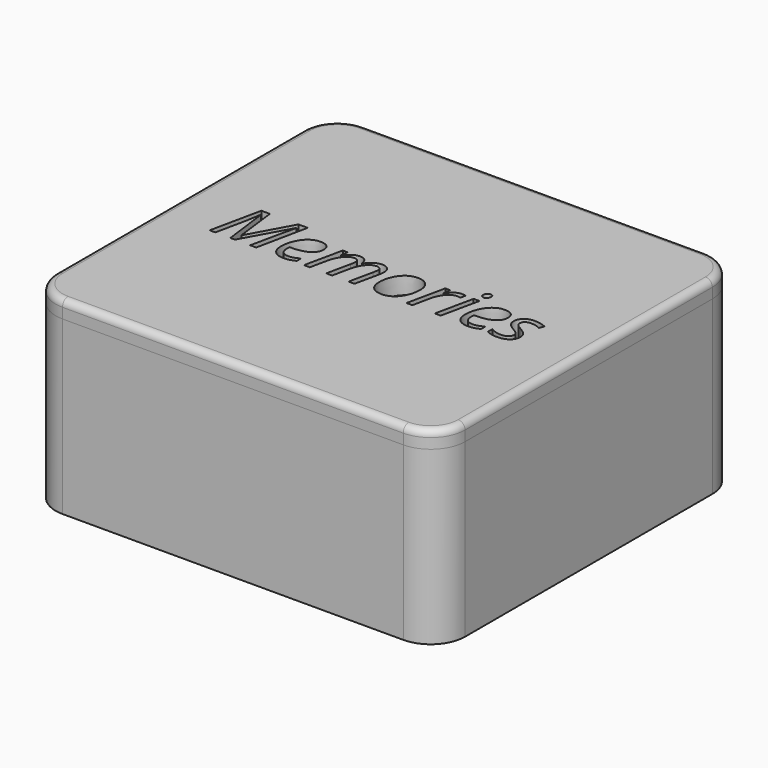
from build123d import *

# Parameters (mm, degrees)
F0_W         = 119.22
F0_H         = 110
F0_W_2       = 109.22
F0_H_2       = 100
F1_DEPTH     = 5
F2_DEPTH     = 45
F3_R         = 5
F4_R         = 10
F6_DEPTH     = 5
F7_DEPTH     = 10
F8_R         = 2
F8_2_R       = 2
F9_TEXT_SIZE = 20.8333333333
F10_DEPTH    = 25
F11_R        = 2


# Not quite as in the source:
# - Text() gives the source's letters only with a copy of the font that has no kerning and outlines rounded to 1/6400 em; it was checked with that copy


with BuildPart() as f1:
    # F0 (on Top) → F1 (new body)
    with BuildSketch(Plane.XY):
        Rectangle(F0_W, F0_H)
        Rectangle(F0_W_2, F0_H_2, mode=Mode.SUBTRACT)
        Rectangle(F0_W_2, F0_H_2)
    extrude(amount=-F1_DEPTH)

    # F0 (on Top) → F2 (join)
    with BuildSketch(Plane.XY):
        Rectangle(F0_W, F0_H)
        Rectangle(F0_W_2, F0_H_2, mode=Mode.SUBTRACT)
    extrude(amount=F2_DEPTH)

    # F3
    f3_edges = [f1.edges().sort_by_distance(p)[0] for p in [
        (-54.61, 50, 22.5),
        (54.61, 50, 22.5),
        (54.61, -50, 22.5),
        (-54.61, -50, 22.5),
    ]]
    fillet(f3_edges, radius=F3_R)

    # F4
    f4_edges = [f1.edges().sort_by_distance(p)[0] for p in [
        (-59.61, -55, 20),
        (59.61, -55, 20),
        (59.61, 55, 20),
        (-59.61, 55, 20),
    ]]
    fillet(f4_edges, radius=F4_R)

    # F8
    f8_edges = [f1.edges().sort_by_distance(p)[0] for p in [
        (-54.61, 0, 45),
    ]]
    fillet(f8_edges, radius=F8_R)


with BuildPart() as f6:
    # F5 (on face) → F6 (new body)
    with BuildSketch(Plane.XY.offset(45)):
        with BuildLine():
            Line((-59.61, 45), (-59.61, -45))
            ThreePointArc((-59.61, -45), (-56.6810678119, -52.0710678119), (-49.61, -55))
            Line((-49.61, -55), (49.61, -55))
            ThreePointArc((49.61, -55), (56.6810678119, -52.0710678119), (59.61, -45))
            Line((59.61, -45), (59.61, 45))
            ThreePointArc((59.61, 45), (56.6810678119, 52.0710678119), (49.61, 55))
            Line((49.61, 55), (-49.61, 55))
            ThreePointArc((-49.61, 55), (-56.6810678119, 52.0710678119), (-59.61, 45))
        make_face()
        with BuildLine():
            ThreePointArc((54.61, -45), (53.1455339059, -48.5355339059), (49.61, -50))
            Line((49.61, -50), (-49.61, -50))
            ThreePointArc((-49.61, -50), (-53.1455339059, -48.5355339059), (-54.61, -45))
            Line((-54.61, -45), (-54.61, 45))
            ThreePointArc((-54.61, 45), (-53.1455339059, 48.5355339059), (-49.61, 50))
            Line((-49.61, 50), (49.61, 50))
            ThreePointArc((49.61, 50), (53.1455339059, 48.5355339059), (54.61, 45))
            Line((54.61, 45), (54.61, -45))
        make_face(mode=Mode.SUBTRACT)
        with BuildLine():
            Line((-49.61, -50), (49.61, -50))
            ThreePointArc((49.61, -50), (53.1455339059, -48.5355339059), (54.61, -45))
            Line((54.61, -45), (54.61, 45))
            ThreePointArc((54.61, 45), (53.1455339059, 48.5355339059), (49.61, 50))
            Line((49.61, 50), (-49.61, 50))
            ThreePointArc((-49.61, 50), (-53.1455339059, 48.5355339059), (-54.61, 45))
            Line((-54.61, 45), (-54.61, -45))
            ThreePointArc((-54.61, -45), (-53.1455339059, -48.5355339059), (-49.61, -50))
        make_face()
        with BuildLine():
            ThreePointArc((-49.61, -49.5), (-52.7919805153, -48.1819805153), (-54.11, -45))
            Line((-54.11, -45), (-54.11, 45))
            ThreePointArc((-54.11, 45), (-52.7919805153, 48.1819805153), (-49.61, 49.5))
            Line((-49.61, 49.5), (49.61, 49.5))
            ThreePointArc((49.61, 49.5), (52.7919805153, 48.1819805153), (54.11, 45))
            Line((54.11, 45), (54.11, -45))
            ThreePointArc((54.11, -45), (52.7919805153, -48.1819805153), (49.61, -49.5))
            Line((49.61, -49.5), (-49.61, -49.5))
        make_face(mode=Mode.SUBTRACT)
        with BuildLine():
            Line((-54.11, 45), (-54.11, -45))
            ThreePointArc((-54.11, -45), (-52.7919805153, -48.1819805153), (-49.61, -49.5))
            Line((-49.61, -49.5), (49.61, -49.5))
            ThreePointArc((49.61, -49.5), (52.7919805153, -48.1819805153), (54.11, -45))
            Line((54.11, -45), (54.11, 45))
            ThreePointArc((54.11, 45), (52.7919805153, 48.1819805153), (49.61, 49.5))
            Line((49.61, 49.5), (-49.61, 49.5))
            ThreePointArc((-49.61, 49.5), (-52.7919805153, 48.1819805153), (-54.11, 45))
        make_face()
        with BuildLine():
            ThreePointArc((-49.61, -47), (-51.0242135624, -46.4142135624), (-51.61, -45))
            Line((-51.61, -45), (-51.61, 45))
            ThreePointArc((-51.61, 45), (-51.0242135624, 46.4142135624), (-49.61, 47))
            Line((-49.61, 47), (49.61, 47))
            ThreePointArc((49.61, 47), (51.0242135624, 46.4142135624), (51.61, 45))
            Line((51.61, 45), (51.61, -45))
            ThreePointArc((51.61, -45), (51.0242135624, -46.4142135624), (49.61, -47))
            Line((49.61, -47), (-49.61, -47))
        make_face(mode=Mode.SUBTRACT)
        with BuildLine():
            Line((-51.61, 45), (-51.61, -45))
            ThreePointArc((-51.61, -45), (-51.0242135624, -46.4142135624), (-49.61, -47))
            Line((-49.61, -47), (49.61, -47))
            ThreePointArc((49.61, -47), (51.0242135624, -46.4142135624), (51.61, -45))
            Line((51.61, -45), (51.61, 45))
            ThreePointArc((51.61, 45), (51.0242135624, 46.4142135624), (49.61, 47))
            Line((49.61, 47), (-49.61, 47))
            ThreePointArc((-49.61, 47), (-51.0242135624, 46.4142135624), (-51.61, 45))
        make_face()
    extrude(amount=F6_DEPTH)

    # F5 (on face) → F7 (join)
    with BuildSketch(Plane.XY.offset(45)):
        with BuildLine():
            Line((-54.11, 45), (-54.11, -45))
            ThreePointArc((-54.11, -45), (-52.7919805153, -48.1819805153), (-49.61, -49.5))
            Line((-49.61, -49.5), (49.61, -49.5))
            ThreePointArc((49.61, -49.5), (52.7919805153, -48.1819805153), (54.11, -45))
            Line((54.11, -45), (54.11, 45))
            ThreePointArc((54.11, 45), (52.7919805153, 48.1819805153), (49.61, 49.5))
            Line((49.61, 49.5), (-49.61, 49.5))
            ThreePointArc((-49.61, 49.5), (-52.7919805153, 48.1819805153), (-54.11, 45))
        make_face()
        with BuildLine():
            ThreePointArc((-49.61, -47), (-51.0242135624, -46.4142135624), (-51.61, -45))
            Line((-51.61, -45), (-51.61, 45))
            ThreePointArc((-51.61, 45), (-51.0242135624, 46.4142135624), (-49.61, 47))
            Line((-49.61, 47), (49.61, 47))
            ThreePointArc((49.61, 47), (51.0242135624, 46.4142135624), (51.61, 45))
            Line((51.61, 45), (51.61, -45))
            ThreePointArc((51.61, -45), (51.0242135624, -46.4142135624), (49.61, -47))
            Line((49.61, -47), (-49.61, -47))
        make_face(mode=Mode.SUBTRACT)
    extrude(amount=-F7_DEPTH)

    # F8#2
    f8_2_edges = [f6.edges().sort_by_distance(p)[0] for p in [
        (-54.11, 0, 45),
        (-51.61, 0, 45),
    ]]
    fillet(f8_2_edges, radius=F8_2_R)

    # F9 (on face) → F10 (cut)
    with BuildSketch(Plane.XY.offset(50)):
        with Locations((-45.6168619792, -7.5)):
            Text('Memories', F9_TEXT_SIZE, font='Open Sans', font_style=FontStyle.ITALIC, text_align=(TextAlign.LEFT, TextAlign.BOTTOM))
        with BuildLine():
            add(Edge.make_bspline(
                [(-20.5973307292, 2.0426432292), (-20.9684244792, 2.3990885417), (-21.7626953125, 2.3990885417)],
                knots=[0, 0, 0, 1, 1, 1], degree=2))
            add(Edge.make_bspline(
                [(-21.7626953125, 2.3990885417), (-22.8108723958, 2.3990885417), (-23.7320963542, 1.4420572917)],
                knots=[0, 0, 0, 1, 1, 1], degree=2))
            add(Edge.make_bspline(
                [(-23.7320963542, 1.4420572917), (-24.6533203125, 0.4850260417), (-25.1416015625, -1.2141927083)],
                knots=[0, 0, 0, 1, 1, 1], degree=2))
            Line((-25.1416015625, -1.2141927083), (-25.0179036458, -1.2141927083))
            add(Edge.make_bspline(
                [(-25.0179036458, -1.2141927083), (-22.7001953125, -1.2141927083), (-21.4632161458, -0.6087239583)],
                knots=[0, 0, 0, 1, 1, 1], degree=2))
            add(Edge.make_bspline(
                [(-21.4632161458, -0.6087239583), (-20.2262369792, -0.0032552083), (-20.2262369792, 1.1458333333)],
                knots=[0, 0, 0, 1, 1, 1], degree=2))
            add(Edge.make_bspline(
                [(-20.2262369792, 1.1458333333), (-20.2262369792, 1.6861979167), (-20.5973307292, 2.0426432292)],
                knots=[0, 0, 0, 1, 1, 1], degree=2))
        make_face()
        with BuildLine():
            add(Edge.make_bspline(
                [(8.7272135417, -3.3951822917), (9.2008463542, -2.0279947917), (9.2008463542, -0.2669270833)],
                knots=[0, 0, 0, 1, 1, 1], degree=2))
            add(Edge.make_bspline(
                [(9.2008463542, -0.2669270833), (9.2008463542, 0.9016927083), (8.564453125, 1.6292317708)],
                knots=[0, 0, 0, 1, 1, 1], degree=2))
            add(Edge.make_bspline(
                [(8.564453125, 1.6292317708), (7.9280598958, 2.3567708333), (6.8408203125, 2.3567708333)],
                knots=[0, 0, 0, 1, 1, 1], degree=2))
            add(Edge.make_bspline(
                [(6.8408203125, 2.3567708333), (5.7307942708, 2.3567708333), (4.8518880208, 1.6048177083)],
                knots=[0, 0, 0, 1, 1, 1], degree=2))
            add(Edge.make_bspline(
                [(4.8518880208, 1.6048177083), (3.9729817708, 0.8528645833), (3.4895833333, -0.4850260417)],
                knots=[0, 0, 0, 1, 1, 1], degree=2))
            add(Edge.make_bspline(
                [(3.4895833333, -0.4850260417), (3.0061848958, -1.8229166667), (3.0061848958, -3.4602864583)],
                knots=[0, 0, 0, 1, 1, 1], degree=2))
            add(Edge.make_bspline(
                [(3.0061848958, -3.4602864583), (3.0061848958, -4.794921875), (3.65234375, -5.5224609375)],
                knots=[0, 0, 0, 1, 1, 1], degree=2))
            add(Edge.make_bspline(
                [(3.65234375, -5.5224609375), (4.2985026042, -6.25), (5.5094401042, -6.25)],
                knots=[0, 0, 0, 1, 1, 1], degree=2))
            add(Edge.make_bspline(
                [(5.5094401042, -6.25), (6.5673828125, -6.25), (7.4104817708, -5.5061848958)],
                knots=[0, 0, 0, 1, 1, 1], degree=2))
            add(Edge.make_bspline(
                [(7.4104817708, -5.5061848958), (8.2535807292, -4.7623697917), (8.7272135417, -3.3951822917)],
                knots=[0, 0, 0, 1, 1, 1], degree=2))
        make_face()
        with BuildLine():
            add(Edge.make_bspline(
                [(33.0712890625, 2.0426432292), (32.7001953125, 2.3990885417), (31.9059244792, 2.3990885417)],
                knots=[0, 0, 0, 1, 1, 1], degree=2))
            add(Edge.make_bspline(
                [(31.9059244792, 2.3990885417), (30.8577473958, 2.3990885417), (29.9365234375, 1.4420572917)],
                knots=[0, 0, 0, 1, 1, 1], degree=2))
            add(Edge.make_bspline(
                [(29.9365234375, 1.4420572917), (29.0152994792, 0.4850260417), (28.5270182292, -1.2141927083)],
                knots=[0, 0, 0, 1, 1, 1], degree=2))
            Line((28.5270182292, -1.2141927083), (28.6507161458, -1.2141927083))
            add(Edge.make_bspline(
                [(28.6507161458, -1.2141927083), (30.9684244792, -1.2141927083), (32.2054036458, -0.6087239583)],
                knots=[0, 0, 0, 1, 1, 1], degree=2))
            add(Edge.make_bspline(
                [(32.2054036458, -0.6087239583), (33.4423828125, -0.0032552083), (33.4423828125, 1.1458333333)],
                knots=[0, 0, 0, 1, 1, 1], degree=2))
            add(Edge.make_bspline(
                [(33.4423828125, 1.1458333333), (33.4423828125, 1.6861979167), (33.0712890625, 2.0426432292)],
                knots=[0, 0, 0, 1, 1, 1], degree=2))
        make_face()
    extrude(amount=-F10_DEPTH, mode=Mode.SUBTRACT)

    # F11
    f11_edges = [f6.edges().sort_by_distance(p)[0] for p in [
        (-59.61, 0, 50),
    ]]
    fillet(f11_edges, radius=F11_R)


solid = Compound([f1.part, f6.part])
